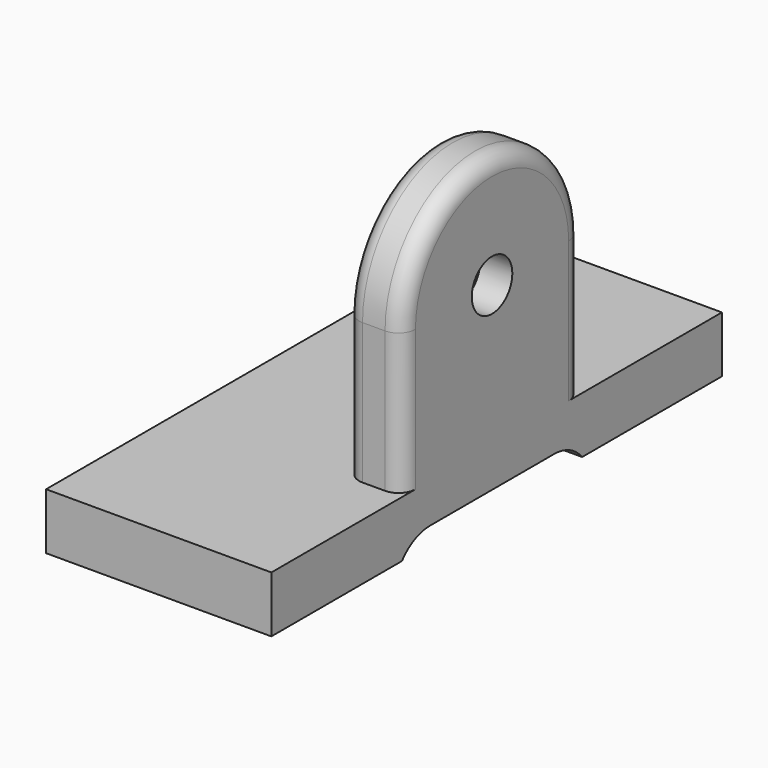
from build123d import *

# Parameters (mm, degrees)
F1_DEPTH     = 10
F3_DEPTH     = 10
F4_R         = 2.25
F5_DEPTH     = 10.001
F6_W         = 40
F6_H         = 3
F7_DEPTH     = 40.001
F8_R         = 4.5
F9_DEPTH     = 5.7
F10_T1_DEPTH = 40
F11_R        = 3


# Not quite as in the source:
# - a fillet or chamfer that OpenCascade refuses, or shapes differently, is made with other operations: its cross-section is extruded or revolved along the edge and cut away or added


with BuildPart() as f1:
    # F0 (on Top) → F1 (new body)
    with BuildSketch(Plane.XY):
        Polygon((0, 100), (0, 0), (40, 0), (40, 96.7579462998), (40, 100), align=None)
    extrude(amount=F1_DEPTH)

    # F2 (on face) → F3 (join)
    with BuildSketch(Plane.YZ.offset(40)):
        with BuildLine():
            Line((28.9808548987, 35), (28.9808548987, 0))
            Line((28.9808548987, 0), (68.9808548987, 0))
            Line((68.9808548987, 0), (68.9808548987, 35))
            ThreePointArc((68.9808548987, 35), (48.9808548987, 55), (28.9808548987, 35))
        make_face()
    extrude(amount=-F3_DEPTH)

    # F4 (on face) → F5 (cut, through all)
    with BuildSketch(Plane(origin=(30, 0, 0), x_dir=(0, -1, 0), z_dir=(-1, 0, 0))):
        with Locations((-48.9808548987, 35)):
            Circle(F4_R)
    extrude(amount=-F5_DEPTH, mode=Mode.SUBTRACT)

    # F6 (on face) → F7 (cut, through all)
    with BuildSketch(Plane.YZ.offset(40)):
        with Locations((48.9808548987, 1.5)):
            Rectangle(F6_W, F6_H)
    extrude(amount=-F7_DEPTH, mode=Mode.SUBTRACT)

    # F8 (on face) → F9 (cut)
    with BuildSketch(Plane.YZ.offset(40)):
        with Locations((48.9808548987, 35)):
            Circle(F8_R)
    extrude(amount=-F9_DEPTH, mode=Mode.SUBTRACT)

    # F10: fillet of radius 8 on 2 edges, made by hand

    # F10_s2 → F10_t1 (join)
    with BuildSketch(Plane.YZ):
        with BuildLine():
            ThreePointArc((68.9808548987, 0), (66.1999585154, 2.2111025509), (62.7358569003, 3))
            Line((62.7358569003, 3), (68.9808548987, 3))
            Line((68.9808548987, 3), (68.9808548987, 0))
        make_face()
        with BuildLine():
            ThreePointArc((35.2258528971, 3), (31.761751282, 2.2111025509), (28.9808548987, 0))
            Line((28.9808548987, 0), (28.9808548987, 3))
            Line((28.9808548987, 3), (35.2258528971, 3))
        make_face()
    extrude(amount=F10_T1_DEPTH)

    # F11
    f11_edges = [f1.edges().sort_by_distance(p)[0] for p in [
        (40, 68.980855, 22.5),
        (30, 68.980855, 22.5),
        (40, 28.980855, 22.5),
        (40, 48.980855, 55),
        (30, 48.980855, 55),
        (30, 28.980855, 22.5),
    ]]
    fillet(f11_edges, radius=F11_R)


solid = f1.part
